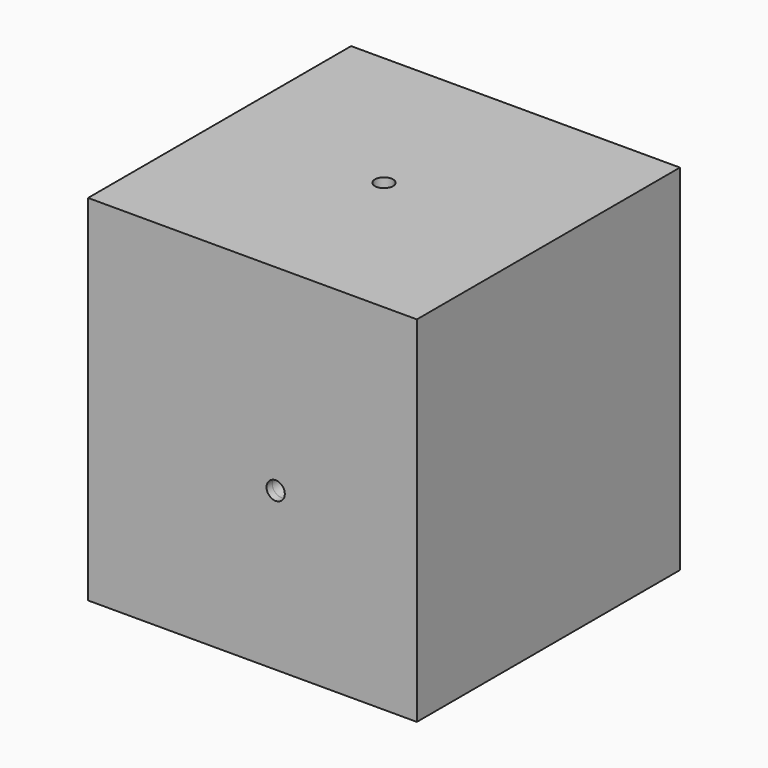
from build123d import *
from build123d import SkipClean  # not in build123d's __all__

# Parameters (mm, degrees)
F0_W     = 90
F0_H     = 90
F0_W_2   = 86
F0_H_2   = 86
F1_DEPTH = 97
F2_W     = 86
F2_H     = 86
F2_R     = 4
F3_DEPTH = 2
F7_R     = 2.5
F8_DEPTH = 76.2


with BuildPart() as f1:
    # F0 (on Top) → F1 (new body)
    with BuildSketch(Plane.XY):
        Rectangle(F0_W, F0_H)
        Rectangle(F0_W_2, F0_H_2, mode=Mode.SUBTRACT)
    extrude(amount=F1_DEPTH)

    # F2 (on face) → F3 (join)
    with BuildSketch(Plane.XY.offset(97)):
        Rectangle(F2_W, F2_H)
        Circle(F2_R, mode=Mode.SUBTRACT)
    extrude(amount=-F3_DEPTH)

    # F4 (on Front) → F6 (revolve)
    with BuildSketch(Plane.XZ):
        Polygon((-2.5, 97), (-4, 97), (-4, 95), (-4, 93.5), (-4.4, 93.5), (-4, 90), (-4.4, 90), (-4, 86.5), (-2.5, 86.5), align=None)
    revolve(axis=Axis((0, 0, 51.8437661231), (0, 0, 1)))

    # F7 (on Front) → F8 (cut)
    with BuildSketch(Plane.XZ):
        with Locations((6.35, 43.18)):
            Circle(F7_R)
    extrude(amount=F8_DEPTH, mode=Mode.SUBTRACT)

    # F11 (on offset) → F12 (revolve)
    with BuildSketch(Plane.YZ.offset(6.35)):
        Polygon((-39.5560968816, 47.18), (-43.0560968816, 47.18), (-43.0560968816, 45.68), (-32.5560968816, 45.68), (-32.5560968816, 47.18), (-36.0560968816, 47.18), align=None)
        Polygon((-39.5560968816, 47.58), (-39.5560968816, 47.18), (-36.0560968816, 47.18), align=None)
        Polygon((-36.0560968816, 47.58), (-36.0560968816, 47.18), (-32.5560968816, 47.18), align=None)
    with SkipClean():  # cleaning this boolean's faces spoils the solid; the shape is the same uncleaned
        revolve(axis=Axis((6.35, -16.5081392042, 43.18), (0, 1, 0)))


solid = f1.part
